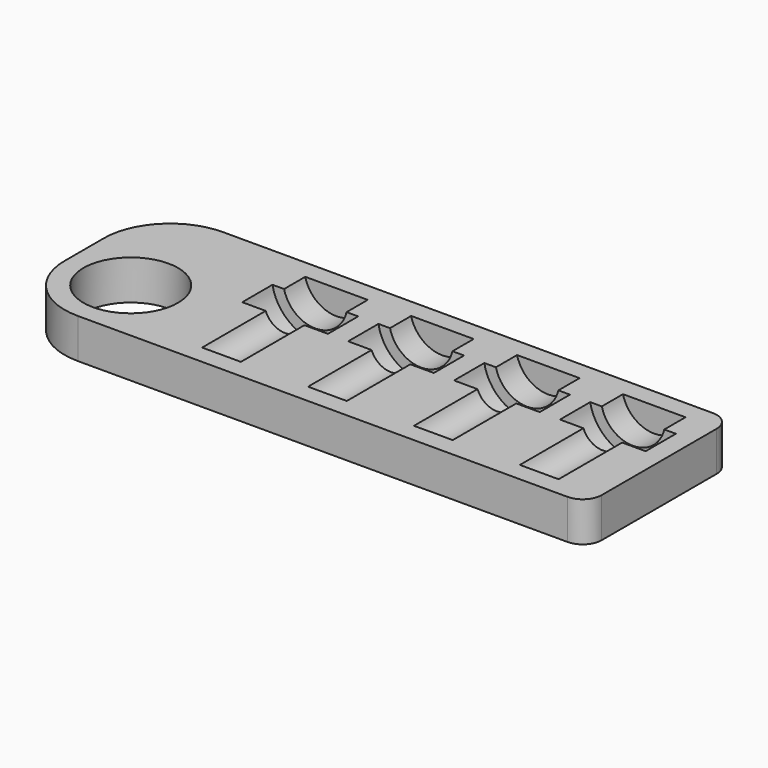
from build123d import *

# Parameters (mm, degrees)
F0_R         = 12.5
F1_DEPTH     = 10.5
F8_TEXT_SIZE = 5.5555555556
F9_DEPTH     = 1


# Not quite as in the source:
# - Text() gives the source's letters only with a copy of the font that has no kerning and outlines rounded to 1/6400 em; it was checked with that copy


with BuildPart() as f1:
    # F0 (on Top) → F1 (new body)
    with BuildSketch(Plane.XY):
        with BuildLine():
            ThreePointArc((0, 17.5), (5.1256313292, 5.1256313292), (17.5, 0))
            Line((17.5, 0), (147, 0))
            ThreePointArc((147, 0), (150.5355339059, 1.4644660941), (152, 5))
            Line((152, 5), (152, 43))
            ThreePointArc((152, 43), (150.5355339059, 46.5355339059), (147, 48))
            Line((147, 48), (17.5, 48))
            ThreePointArc((17.5, 48), (5.1256313292, 42.8743686708), (0, 30.5))
            Line((0, 30.5), (0, 17.5))
        make_face()
        with Locations((17.5, 17.5)):
            Circle(F0_R, mode=Mode.SUBTRACT)
    extrude(amount=F1_DEPTH)

    # F3 (on offset) → F4 (revolve, cut)
    with BuildSketch(Plane.XY.offset(12.5)):
        Polygon((51.5, 26), (51.5, 5), (57, 5), (57, 26), (63, 26), (63, 36), (60, 36), (60, 43), (51.5, 43), (51.5, 36), align=None)
    revolve(axis=Axis((51.5, 31, 12.5), (0, 1, 0)), mode=Mode.SUBTRACT)

    # F3 (on offset) → F5 (revolve, cut)
    with BuildSketch(Plane.XY.offset(12.5)):
        Polygon((79.5, 26), (79.5, 5), (85, 5), (85, 26), (91, 26), (91, 36), (88, 36), (88, 43), (79.5, 43), (79.5, 36), align=None)
    revolve(axis=Axis((79.5, 31, 12.5), (0, 1, 0)), mode=Mode.SUBTRACT)

    # F3 (on offset) → F6 (revolve, cut)
    with BuildSketch(Plane.XY.offset(12.5)):
        Polygon((107.5, 26), (107.5, 5), (113, 5), (113, 26), (119, 26), (119, 36), (116, 36), (116, 43), (107.5, 43), (107.5, 36), align=None)
    revolve(axis=Axis((107.5, 31, 12.5), (0, 1, 0)), mode=Mode.SUBTRACT)

    # F3 (on offset) → F7 (revolve, cut)
    with BuildSketch(Plane.XY.offset(12.5)):
        Polygon((135.5, 26), (135.5, 5), (141, 5), (141, 26), (147, 26), (147, 36), (144, 36), (144, 43), (135.5, 43), (135.5, 36), align=None)
    revolve(axis=Axis((135.5, 31, 12.5), (0, 1, 0)), mode=Mode.SUBTRACT)

    # F8 (on face) → F9 (cut)
    with BuildSketch(Plane(origin=(0, 0, 0), x_dir=(1, 0, 0), z_dir=(0, 0, -1))):
        with Locations((30, -9)):
            Text('810, 811', F8_TEXT_SIZE, font='Open Sans', text_align=(TextAlign.LEFT, TextAlign.BOTTOM))
    extrude(amount=-F9_DEPTH, mode=Mode.SUBTRACT)


solid = f1.part
